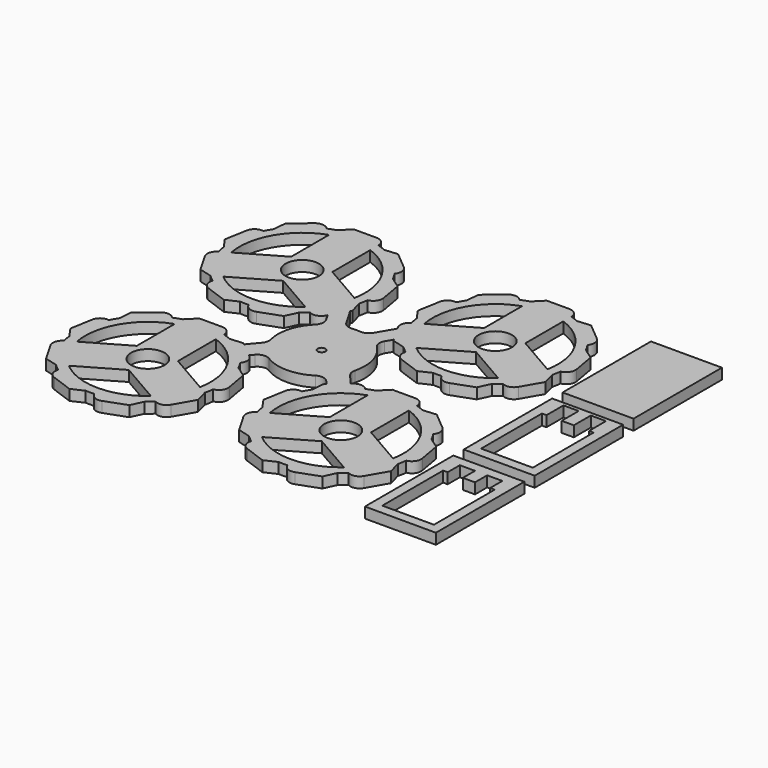
from build123d import *

# Parameters (mm, degrees)
F0_R     = 11
F0_R_2   = 2.5527
F1_DEPTH = 7
F0_W     = 46.7
F0_H     = 72.7


# Not quite as in the source:
# - a feature names something its author has since deleted; it is built from what else it names


with BuildPart() as f1:
    # F0 (on Top) → F1 (new body)
    with BuildSketch(Plane.XY):
        with BuildLine():
            Line((-7.4638039729, 51.7525), (-13.5636, 45.6527039729))
            ThreePointArc((-13.5636, 45.6527039729), (-16.2887093259, 44.7528610649), (-18.9546720538, 43.6905142146))
            ThreePointArc((-18.9546720538, 43.6905142146), (-23.0957546511, 45.8462253684), (-27.5482602123, 44.4423557574))
            Line((-27.5482602123, 44.4423557574), (-38.9834713283, 34.8470743276))
            Line((-38.9834713283, 34.8470743276), (-39.7353128712, 26.2534861691))
            ThreePointArc((-39.7353128712, 26.2534861691), (-41.2444598552, 23.8125), (-42.6038423959, 21.2850472892))
            ThreePointArc((-42.6038423959, 21.2850472892), (-47.1617601278, 20.2745812553), (-49.6701872794, 16.3371393342))
            Line((-49.6701872794, 16.3371393342), (-52.2623391961, 1.6363152952))
            Line((-52.2623391961, 1.6363152952), (-47.3144312411, -5.4300295883))
            ThreePointArc((-47.3144312411, -5.4300295883), (-46.9014692372, -8.2699944614), (-46.318201392, -11.0799298197))
            ThreePointArc((-46.318201392, -11.0799298197), (-49.1602538961, -14.783764754), (-48.5508816958, -19.4124061506))
            Line((-48.5508816958, -19.4124061506), (-41.0870777229, -32.3400938494))
            Line((-41.0870777229, -32.3400938494), (-32.754601392, -34.5727741532))
            ThreePointArc((-32.754601392, -34.5727741532), (-30.6127599113, -36.4828666035), (-28.3597591873, -38.2604846263))
            ThreePointArc((-28.3597591873, -38.2604846263), (-28.156118511, -42.9246229316), (-24.7140789838, -46.0786710526))
            Line((-24.7140789838, -46.0786710526), (-10.6867159511, -51.1842136618))
            Line((-10.6867159511, -51.1842136618), (-2.8685295247, -47.5385334583))
            ThreePointArc((-2.8685295247, -47.5385334583), (0, -47.625), (2.8685295247, -47.5385334583))
            ThreePointArc((2.8685295247, -47.5385334583), (6.0225776457, -50.9805729855), (10.6867159511, -51.1842136618))
            Line((10.6867159511, -51.1842136618), (24.7140789838, -46.0786710526))
            Line((24.7140789838, -46.0786710526), (28.3597591873, -38.2604846263))
            ThreePointArc((28.3597591873, -38.2604846263), (30.6127599113, -36.4828666035), (32.754601392, -34.5727741532))
            ThreePointArc((32.754601392, -34.5727741532), (37.3832427886, -35.1821463535), (41.0870777229, -32.3400938494))
            Line((41.0870777229, -32.3400938494), (41.7220777229, -31.2402415866))
            Line((41.7220777229, -31.2402415866), (44.2734834239, -35.6594058915))
            ThreePointArc((44.2734834239, -35.6594058915), (45.0704007857, -39.6594113953), (43.2698180899, -43.3190593657))
            ThreePointArc((43.2698180899, -43.3190593657), (35.9384869045, -55.9572139837), (35.8127567766, -70.5673324307))
            ThreePointArc((35.8127567766, -70.5673324307), (35.8512424012, -73.5490431677), (34.524418274, -76.2195520701))
            Line((34.524418274, -76.2195520701), (28.5211366551, -83.3739845069))
            Line((28.5211366551, -83.3739845069), (27.5482602123, -82.5576442426))
            Line((27.5482602123, -82.5576442426), (18.9546720538, -83.3094857854))
            ThreePointArc((18.9546720538, -83.3094857854), (16.2887093259, -82.2471389351), (13.5636, -81.3472960271))
            ThreePointArc((13.5636, -81.3472960271), (11.7770111075, -77.0340888925), (7.4638039729, -75.2475))
            Line((7.4638039729, -75.2475), (-7.4638039729, -75.2475))
            Line((-7.4638039729, -75.2475), (-13.5636, -81.3472960271))
            ThreePointArc((-13.5636, -81.3472960271), (-16.2887093259, -82.2471389351), (-18.9546720538, -83.3094857854))
            ThreePointArc((-18.9546720538, -83.3094857854), (-23.0957546511, -81.1537746316), (-27.5482602123, -82.5576442426))
            Line((-27.5482602123, -82.5576442426), (-38.9834713283, -92.1529256724))
            Line((-38.9834713283, -92.1529256724), (-39.7353128712, -100.7465138309))
            ThreePointArc((-39.7353128712, -100.7465138309), (-41.2444598552, -103.1875), (-42.6038423959, -105.7149527108))
            ThreePointArc((-42.6038423959, -105.7149527108), (-47.1617601278, -106.7254187447), (-49.6701872794, -110.6628606658))
            Line((-49.6701872794, -110.6628606658), (-52.2623391961, -125.3636847048))
            Line((-52.2623391961, -125.3636847048), (-47.3144312411, -132.4300295883))
            ThreePointArc((-47.3144312411, -132.4300295883), (-46.9014692372, -135.2699944614), (-46.318201392, -138.0799298197))
            ThreePointArc((-46.318201392, -138.0799298197), (-49.1602538961, -141.783764754), (-48.5508816958, -146.4124061506))
            Line((-48.5508816958, -146.4124061506), (-41.0870777229, -159.3400938494))
            Line((-41.0870777229, -159.3400938494), (-32.754601392, -161.5727741532))
            ThreePointArc((-32.754601392, -161.5727741532), (-30.6127599113, -163.4828666035), (-28.3597591873, -165.2604846263))
            ThreePointArc((-28.3597591873, -165.2604846263), (-28.156118511, -169.9246229316), (-24.7140789838, -173.0786710526))
            Line((-24.7140789838, -173.0786710526), (-10.6867159511, -178.1842136618))
            Line((-10.6867159511, -178.1842136618), (-2.8685295247, -174.5385334583))
            ThreePointArc((-2.8685295247, -174.5385334583), (0, -174.625), (2.8685295247, -174.5385334583))
            ThreePointArc((2.8685295247, -174.5385334583), (6.0225776457, -177.9805729855), (10.6867159511, -178.1842136618))
            Line((10.6867159511, -178.1842136618), (24.7140789838, -173.0786710526))
            Line((24.7140789838, -173.0786710526), (28.3597591873, -165.2604846263))
            ThreePointArc((28.3597591873, -165.2604846263), (30.6127599113, -163.4828666035), (32.754601392, -161.5727741532))
            ThreePointArc((32.754601392, -161.5727741532), (37.3832427886, -162.1821463535), (41.0870777229, -159.3400938494))
            Line((41.0870777229, -159.3400938494), (48.5508816958, -146.4124061506))
            Line((48.5508816958, -146.4124061506), (46.318201392, -138.0799298197))
            ThreePointArc((46.318201392, -138.0799298197), (46.9014692372, -135.2699944614), (47.3144312411, -132.4300295883))
            ThreePointArc((47.3144312411, -132.4300295883), (51.2518731622, -129.9216024367), (52.2623391961, -125.3636847048))
            Line((52.2623391961, -125.3636847048), (49.6701872794, -110.6628606658))
            Line((49.6701872794, -110.6628606658), (42.6038423959, -105.7149527108))
            ThreePointArc((42.6038423959, -105.7149527108), (41.2444598552, -103.1875), (39.7353128712, -100.7465138309))
            ThreePointArc((39.7353128712, -100.7465138309), (41.1391824821, -96.2940082698), (38.9834713283, -92.1529256724))
            Line((38.9834713283, -92.1529256724), (38.0105948855, -91.3365854081))
            Line((38.0105948855, -91.3365854081), (40.0053845071, -88.9592877101))
            ThreePointArc((40.0053845071, -88.9592877101), (43.8894290876, -86.7671195618), (48.2570818626, -87.6699001168))
            ThreePointArc((48.2570818626, -87.6699001168), (63.5, -92.075), (78.7429181374, -87.6699001168))
            ThreePointArc((78.7429181374, -87.6699001168), (83.1105709124, -86.7671195618), (86.9946154929, -88.9592877101))
            Line((86.9946154929, -88.9592877101), (88.9894051145, -91.3365854081))
            Line((88.9894051145, -91.3365854081), (88.0165286717, -92.1529256724))
            Line((88.0165286717, -92.1529256724), (87.2646871288, -100.7465138309))
            ThreePointArc((87.2646871288, -100.7465138309), (85.7555401448, -103.1875), (84.3961576041, -105.7149527108))
            ThreePointArc((84.3961576041, -105.7149527108), (79.8382398722, -106.7254187447), (77.3298127206, -110.6628606658))
            Line((77.3298127206, -110.6628606658), (74.7376608039, -125.3636847048))
            Line((74.7376608039, -125.3636847048), (79.6855687589, -132.4300295883))
            ThreePointArc((79.6855687589, -132.4300295883), (80.0985307628, -135.2699944614), (80.681798608, -138.0799298197))
            ThreePointArc((80.681798608, -138.0799298197), (77.8397461039, -141.783764754), (78.4491183042, -146.4124061506))
            Line((78.4491183042, -146.4124061506), (85.9129222771, -159.3400938494))
            Line((85.9129222771, -159.3400938494), (94.245398608, -161.5727741532))
            ThreePointArc((94.245398608, -161.5727741532), (96.3872400887, -163.4828666035), (98.6402408127, -165.2604846263))
            ThreePointArc((98.6402408127, -165.2604846263), (98.843881489, -169.9246229316), (102.2859210162, -173.0786710526))
            Line((102.2859210162, -173.0786710526), (116.3132840489, -178.1842136618))
            Line((116.3132840489, -178.1842136618), (124.1314704753, -174.5385334583))
            ThreePointArc((124.1314704753, -174.5385334583), (127, -174.625), (129.8685295247, -174.5385334583))
            ThreePointArc((129.8685295247, -174.5385334583), (133.0225776457, -177.9805729855), (137.6867159511, -178.1842136618))
            Line((137.6867159511, -178.1842136618), (151.7140789838, -173.0786710526))
            Line((151.7140789838, -173.0786710526), (155.3597591873, -165.2604846263))
            ThreePointArc((155.3597591873, -165.2604846263), (157.6127599113, -163.4828666035), (159.754601392, -161.5727741532))
            ThreePointArc((159.754601392, -161.5727741532), (164.3832427886, -162.1821463535), (168.0870777229, -159.3400938494))
            Line((168.0870777229, -159.3400938494), (175.5508816958, -146.4124061506))
            Line((175.5508816958, -146.4124061506), (173.318201392, -138.0799298197))
            ThreePointArc((173.318201392, -138.0799298197), (173.9014692372, -135.2699944614), (174.3144312411, -132.4300295883))
            ThreePointArc((174.3144312411, -132.4300295883), (178.2518731622, -129.9216024367), (179.2623391961, -125.3636847048))
            Line((179.2623391961, -125.3636847048), (176.6701872794, -110.6628606658))
            Line((176.6701872794, -110.6628606658), (169.6038423959, -105.7149527108))
            ThreePointArc((169.6038423959, -105.7149527108), (168.2444598552, -103.1875), (166.7353128712, -100.7465138309))
            ThreePointArc((166.7353128712, -100.7465138309), (168.1391824821, -96.2940082698), (165.9834713283, -92.1529256724))
            Line((165.9834713283, -92.1529256724), (154.5482602123, -82.5576442426))
            Line((154.5482602123, -82.5576442426), (145.9546720538, -83.3094857854))
            ThreePointArc((145.9546720538, -83.3094857854), (143.2887093259, -82.2471389351), (140.5636, -81.3472960271))
            ThreePointArc((140.5636, -81.3472960271), (138.7770111075, -77.0340888925), (134.4638039729, -75.2475))
            Line((134.4638039729, -75.2475), (119.5361960271, -75.2475))
            Line((119.5361960271, -75.2475), (113.4364, -81.3472960271))
            ThreePointArc((113.4364, -81.3472960271), (110.7112906741, -82.2471389351), (108.0453279462, -83.3094857854))
            ThreePointArc((108.0453279462, -83.3094857854), (103.9042453489, -81.1537746316), (99.4517397877, -82.5576442426))
            Line((99.4517397877, -82.5576442426), (98.4788633449, -83.3739845069))
            Line((98.4788633449, -83.3739845069), (92.475581726, -76.2195520701))
            ThreePointArc((92.475581726, -76.2195520701), (91.1487575988, -73.5490431677), (91.1872432234, -70.5673324307))
            ThreePointArc((91.1872432234, -70.5673324307), (91.0568361681, -55.9401451468), (83.7051681746, -43.294015638))
            ThreePointArc((83.7051681746, -43.294015638), (81.8961741463, -39.6067311446), (82.7223187386, -35.5835469029))
            Line((82.7223187386, -35.5835469029), (85.2779222771, -31.2402415866))
            Line((85.2779222771, -31.2402415866), (85.9129222771, -32.3400938494))
            Line((85.9129222771, -32.3400938494), (94.245398608, -34.5727741532))
            ThreePointArc((94.245398608, -34.5727741532), (96.3872400887, -36.4828666035), (98.6402408127, -38.2604846263))
            ThreePointArc((98.6402408127, -38.2604846263), (98.843881489, -42.9246229316), (102.2859210162, -46.0786710526))
            Line((102.2859210162, -46.0786710526), (116.3132840489, -51.1842136618))
            Line((116.3132840489, -51.1842136618), (124.1314704753, -47.5385334583))
            ThreePointArc((124.1314704753, -47.5385334583), (127, -47.625), (129.8685295247, -47.5385334583))
            ThreePointArc((129.8685295247, -47.5385334583), (133.0225776457, -50.9805729855), (137.6867159511, -51.1842136618))
            Line((137.6867159511, -51.1842136618), (151.7140789838, -46.0786710526))
            Line((151.7140789838, -46.0786710526), (155.3597591873, -38.2604846263))
            ThreePointArc((155.3597591873, -38.2604846263), (157.6127599113, -36.4828666035), (159.754601392, -34.5727741532))
            ThreePointArc((159.754601392, -34.5727741532), (164.3832427886, -35.1821463535), (168.0870777229, -32.3400938494))
            Line((168.0870777229, -32.3400938494), (175.5508816958, -19.4124061506))
            Line((175.5508816958, -19.4124061506), (173.318201392, -11.0799298197))
            ThreePointArc((173.318201392, -11.0799298197), (173.9014692372, -8.2699944614), (174.3144312411, -5.4300295883))
            ThreePointArc((174.3144312411, -5.4300295883), (178.2518731622, -2.9216024367), (179.2623391961, 1.6363152952))
            Line((179.2623391961, 1.6363152952), (176.6701872794, 16.3371393342))
            Line((176.6701872794, 16.3371393342), (169.6038423959, 21.2850472892))
            ThreePointArc((169.6038423959, 21.2850472892), (168.2444598552, 23.8125), (166.7353128712, 26.2534861691))
            ThreePointArc((166.7353128712, 26.2534861691), (168.1391824821, 30.7059917302), (165.9834713283, 34.8470743276))
            Line((165.9834713283, 34.8470743276), (154.5482602123, 44.4423557574))
            Line((154.5482602123, 44.4423557574), (145.9546720538, 43.6905142146))
            ThreePointArc((145.9546720538, 43.6905142146), (143.2887093259, 44.7528610649), (140.5636, 45.6527039729))
            ThreePointArc((140.5636, 45.6527039729), (138.7770111075, 49.9659111075), (134.4638039729, 51.7525))
            Line((134.4638039729, 51.7525), (119.5361960271, 51.7525))
            Line((119.5361960271, 51.7525), (113.4364, 45.6527039729))
            ThreePointArc((113.4364, 45.6527039729), (110.7112906741, 44.7528610649), (108.0453279462, 43.6905142146))
            ThreePointArc((108.0453279462, 43.6905142146), (103.9042453489, 45.8462253684), (99.4517397877, 44.4423557574))
            Line((99.4517397877, 44.4423557574), (88.0165286717, 34.8470743276))
            Line((88.0165286717, 34.8470743276), (87.2646871288, 26.2534861691))
            ThreePointArc((87.2646871288, 26.2534861691), (85.7555401448, 23.8125), (84.3961576041, 21.2850472892))
            ThreePointArc((84.3961576041, 21.2850472892), (79.8382398722, 20.2745812553), (77.3298127206, 16.3371393342))
            Line((77.3298127206, 16.3371393342), (74.7376608039, 1.6363152952))
            Line((74.7376608039, 1.6363152952), (79.6855687589, -5.4300295883))
            ThreePointArc((79.6855687589, -5.4300295883), (80.0985307628, -8.2699944614), (80.681798608, -11.0799298197))
            ThreePointArc((80.681798608, -11.0799298197), (77.8397461039, -14.783764754), (78.4491183042, -19.4124061506))
            Line((78.4491183042, -19.4124061506), (79.0841183042, -20.5122584134))
            Line((79.0841183042, -20.5122584134), (72.3489606045, -31.9588094149))
            ThreePointArc((72.3489606045, -31.9588094149), (69.757934806, -34.3969494029), (66.262242197, -35.0588213492))
            ThreePointArc((66.262242197, -35.0588213492), (63.4509070052, -34.9250421719), (60.6400480849, -35.0684805182))
            ThreePointArc((60.6400480849, -35.0684805182), (57.1090363993, -34.4018048873), (54.5052419008, -31.9253650778))
            Line((54.5052419008, -31.9253650778), (47.9158816958, -20.5122584134))
            Line((47.9158816958, -20.5122584134), (48.5508816958, -19.4124061506))
            Line((48.5508816958, -19.4124061506), (46.318201392, -11.0799298197))
            ThreePointArc((46.318201392, -11.0799298197), (46.9014692372, -8.2699944614), (47.3144312411, -5.4300295883))
            ThreePointArc((47.3144312411, -5.4300295883), (51.2518731622, -2.9216024367), (52.2623391961, 1.6363152952))
            Line((52.2623391961, 1.6363152952), (49.6701872794, 16.3371393342))
            Line((49.6701872794, 16.3371393342), (42.6038423959, 21.2850472892))
            ThreePointArc((42.6038423959, 21.2850472892), (41.2444598552, 23.8125), (39.7353128712, 26.2534861691))
            ThreePointArc((39.7353128712, 26.2534861691), (41.1391824821, 30.7059917302), (38.9834713283, 34.8470743276))
            Line((38.9834713283, 34.8470743276), (27.5482602123, 44.4423557574))
            Line((27.5482602123, 44.4423557574), (18.9546720538, 43.6905142146))
            ThreePointArc((18.9546720538, 43.6905142146), (16.2887093259, 44.7528610649), (13.5636, 45.6527039729))
            ThreePointArc((13.5636, 45.6527039729), (11.7770111075, 49.9659111075), (7.4638039729, 51.7525))
            Line((7.4638039729, 51.7525), (-7.4638039729, 51.7525))
        make_face()
        with BuildLine():
            Line((0, -142.6618962224), (26.9782471716, -158.2377944892))
            ThreePointArc((26.9782471716, -158.2377944892), (0, -168.275), (-26.9782471716, -158.2377944892))
            Line((-26.9782471716, -158.2377944892), (0, -142.6618962224))
        make_face(mode=Mode.SUBTRACT)
        with Locations((0, -127)):
            Circle(F0_R, mode=Mode.SUBTRACT)
        with BuildLine():
            Line((-13.5636, -119.1690518888), (-40.5418471716, -134.7449501556))
            ThreePointArc((-40.5418471716, -134.7449501556), (-35.7451985412, -106.3625), (-13.5636, -88.0172553552))
            Line((-13.5636, -88.0172553552), (-13.5636, -119.1690518888))
        make_face(mode=Mode.SUBTRACT)
        with BuildLine():
            Line((40.5418471716, -134.7449501556), (13.5636, -119.1690518888))
            Line((13.5636, -119.1690518888), (13.5636, -88.0172553552))
            ThreePointArc((13.5636, -88.0172553552), (35.7451985412, -106.3625), (40.5418471716, -134.7449501556))
        make_face(mode=Mode.SUBTRACT)
        with BuildLine():
            Line((127, -142.6618962224), (153.9782471716, -158.2377944892))
            ThreePointArc((153.9782471716, -158.2377944892), (127, -168.275), (100.0217528284, -158.2377944892))
            Line((100.0217528284, -158.2377944892), (127, -142.6618962224))
        make_face(mode=Mode.SUBTRACT)
        with Locations((127, -127)):
            Circle(F0_R, mode=Mode.SUBTRACT)
        with BuildLine():
            Line((113.4364, -119.1690518888), (86.4581528284, -134.7449501556))
            ThreePointArc((86.4581528284, -134.7449501556), (91.2548014588, -106.3625), (113.4364, -88.0172553552))
            Line((113.4364, -88.0172553552), (113.4364, -119.1690518888))
        make_face(mode=Mode.SUBTRACT)
        with BuildLine():
            Line((167.5418471716, -134.7449501556), (140.5636, -119.1690518888))
            Line((140.5636, -119.1690518888), (140.5636, -88.0172553552))
            ThreePointArc((140.5636, -88.0172553552), (162.7451985412, -106.3625), (167.5418471716, -134.7449501556))
        make_face(mode=Mode.SUBTRACT)
        with BuildLine():
            ThreePointArc((26.9782471716, -31.2377944892), (0, -41.275), (-26.9782471716, -31.2377944892))
            Line((-26.9782471716, -31.2377944892), (0, -15.6618962224))
            Line((0, -15.6618962224), (26.9782471716, -31.2377944892))
        make_face(mode=Mode.SUBTRACT)
        with Locations((63.5, -63.5)):
            Circle(F0_R_2, mode=Mode.SUBTRACT)
        with BuildLine():
            ThreePointArc((-40.5418471716, -7.7449501556), (-35.7451985412, 20.6375), (-13.5636, 38.9827446448))
            Line((-13.5636, 38.9827446448), (-13.5636, 7.8309481112))
            Line((-13.5636, 7.8309481112), (-40.5418471716, -7.7449501556))
        make_face(mode=Mode.SUBTRACT)
        Circle(F0_R, mode=Mode.SUBTRACT)
        with BuildLine():
            ThreePointArc((13.5636, 38.9827446448), (35.7451985412, 20.6375), (40.5418471716, -7.7449501556))
            Line((40.5418471716, -7.7449501556), (13.5636, 7.8309481112))
            Line((13.5636, 7.8309481112), (13.5636, 38.9827446448))
        make_face(mode=Mode.SUBTRACT)
        with BuildLine():
            Line((127, -15.6618962224), (153.9782471716, -31.2377944892))
            ThreePointArc((153.9782471716, -31.2377944892), (127, -41.275), (100.0217528284, -31.2377944892))
            Line((100.0217528284, -31.2377944892), (127, -15.6618962224))
        make_face(mode=Mode.SUBTRACT)
        with Locations((127, 0)):
            Circle(F0_R, mode=Mode.SUBTRACT)
        with BuildLine():
            Line((113.4364, 7.8309481112), (86.4581528284, -7.7449501556))
            ThreePointArc((86.4581528284, -7.7449501556), (91.2548014588, 20.6375), (113.4364, 38.9827446448))
            Line((113.4364, 38.9827446448), (113.4364, 7.8309481112))
        make_face(mode=Mode.SUBTRACT)
        with BuildLine():
            Line((167.5418471716, -7.7449501556), (140.5636, 7.8309481112))
            Line((140.5636, 7.8309481112), (140.5636, 38.9827446448))
            ThreePointArc((140.5636, 38.9827446448), (162.7451985412, 20.6375), (167.5418471716, -7.7449501556))
        make_face(mode=Mode.SUBTRACT)
    extrude(amount=F1_DEPTH)


with BuildPart() as f1b:
    # F0 (on Top) → F1, piece 2 (new body)
    with BuildSketch(Plane.XY):
        with Locations((213.0376608039, -149.1975)):
            Rectangle(F0_W, F0_H)
        Polygon((227.0376608039, -119.1975), (227.0376608039, -129.1975), (230.0376608039, -129.1975), (230.0376608039, -179.1975), (196.0376608039, -179.1975), (196.0376608039, -129.1975), (199.0376608039, -129.1975), (199.0376608039, -119.1975), (209.0376662039, -119.1975), (209.0376662039, -129.1975), (217.0376608039, -129.1975), (217.0376608039, -119.1975), align=None, mode=Mode.SUBTRACT)
    extrude(amount=F1_DEPTH)


with BuildPart() as f1c:
    # F0 (on Top) → F1, piece 3 (new body)
    with BuildSketch(Plane.XY):
        with Locations((213.0376608039, -67.9175)):
            Rectangle(F0_W, F0_H)
        Polygon((230.0376608039, -97.9175), (196.0376608039, -97.9175), (196.0376608039, -47.9175), (199.0376608039, -47.9175), (199.0376608039, -37.9175), (199.0376608039, -33.9475), (209.0376662039, -33.9475), (209.0376662039, -37.9175), (209.0376662039, -47.9175), (217.0376608039, -47.9175), (217.0376608039, -37.9175), (217.0376608039, -33.9475), (227.0211577415, -33.9475), (227.0211577415, -37.9175), (227.0376608039, -37.9175), (227.0376608039, -47.9175), (230.0376608039, -47.9175), align=None, mode=Mode.SUBTRACT)
    extrude(amount=F1_DEPTH)


with BuildPart() as f1d:
    # F0 (on Top) → F1, piece 4 (new body)
    with BuildSketch(Plane.XY):
        Polygon((236.3876608039, -22.9875), (236.3876608039, 49.7125), (227.2822856903, 49.7125), (227.2822856903, 43.3625), (227.0376608039, 43.3625), (227.0376608039, 33.3625), (230.0376608039, 33.3625), (230.0376608039, -16.6375), (196.0376608039, -16.6375), (196.0376608039, 33.3625), (199.0376608039, 33.3625), (199.0376608039, 43.3625), (199.0376608039, 49.7125), (189.6876608039, 49.7125), (189.6876608039, -22.9875), align=None)
        Polygon((227.2822856903, 43.3625), (227.2822856903, 49.7125), (217.0376608039, 49.7125), (217.0376608039, 43.3625), (217.0376608039, 33.3625), (209.0376662039, 33.3625), (209.0376662039, 43.3625), (209.0376662039, 49.7125), (199.0376608039, 49.7125), (199.0376608039, 43.3625), (199.0376608039, 33.3625), (196.0376608039, 33.3625), (196.0376608039, -16.6375), (230.0376608039, -16.6375), (230.0376608039, 33.3625), (227.0376608039, 33.3625), (227.0376608039, 43.3625), align=None)
        Polygon((217.0376608039, 43.3625), (217.0376608039, 49.7125), (209.0376662039, 49.7125), (209.0376662039, 43.3625), (209.0376662039, 33.3625), (217.0376608039, 33.3625), align=None)
    extrude(amount=F1_DEPTH)


solid = Compound([f1.part, f1b.part, f1c.part, f1d.part])
